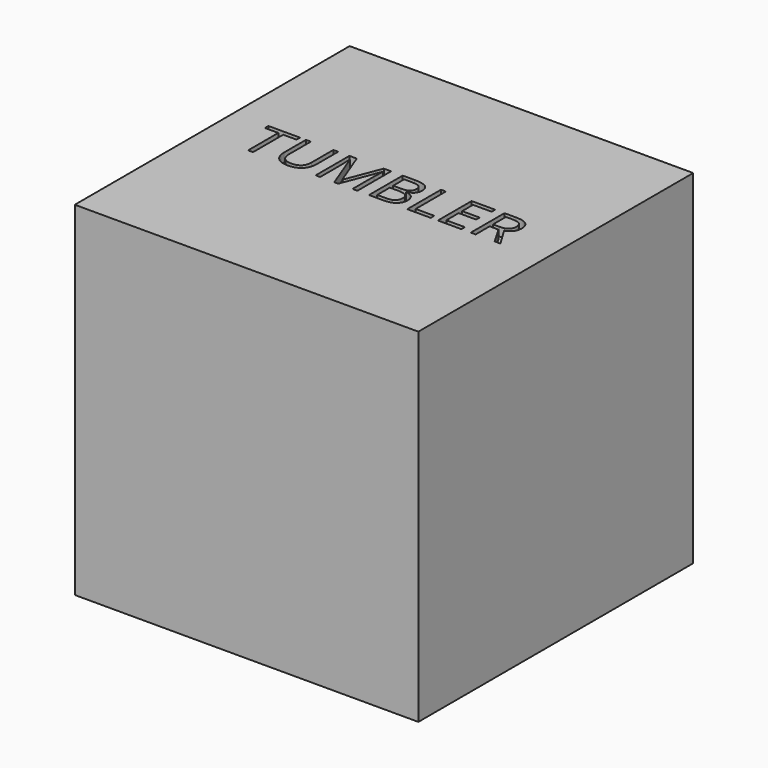
from build123d import *

# Parameters (mm, degrees)
F0_W         = 1000
F0_H         = 1000
F1_DEPTH     = 1000
F2_TEXT_SIZE = 171.8889349516
F3_DEPTH     = 25


# Not quite as in the source:
# - Text() gives the source's letters only with a copy of the font that has no kerning and outlines rounded to 1/6400 em; it was checked with that copy


with BuildPart() as f1:
    # F0 (on Top) → F1 (new body)
    with BuildSketch(Plane.XY):
        Rectangle(F0_W, F0_H)
    extrude(amount=F1_DEPTH)

    # F2 (on face) → F3 (cut)
    with BuildSketch(Plane.XY.offset(1000)):
        with Locations((-400, -45.0566958815)):
            Text('TUMBLER', F2_TEXT_SIZE, font='Open Sans', text_align=(TextAlign.LEFT, TextAlign.BOTTOM))
    extrude(amount=-F3_DEPTH, mode=Mode.SUBTRACT)


solid = f1.part
